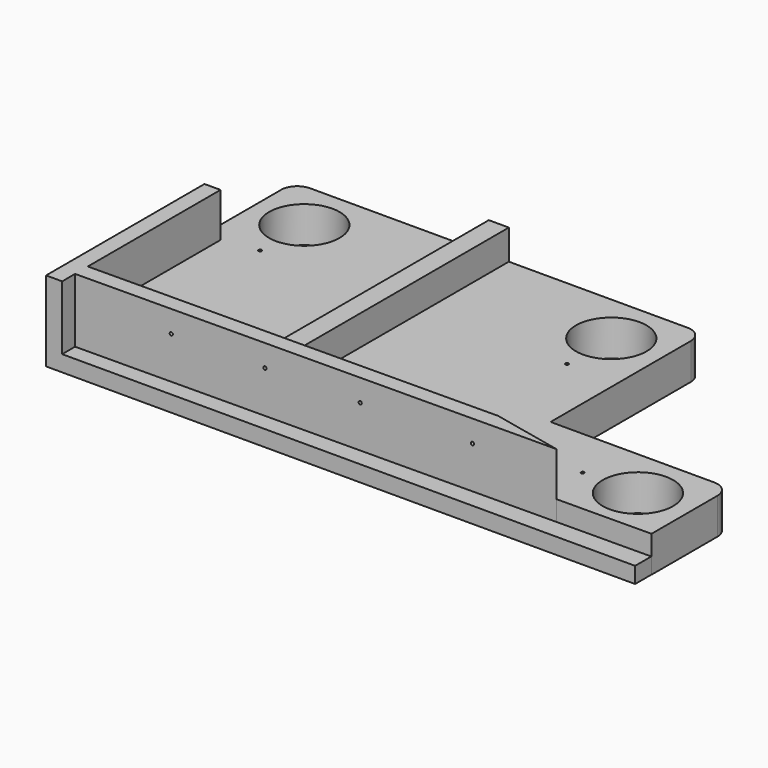
from build123d import *

# Parameters (mm, degrees)
F0_R      = 0.508
F0_R_2    = 11.176
F1_DEPTH  = 11.43
F3_DEPTH  = 25.4
F4_R      = 0.508
F5_DEPTH  = 11.4608454435
F6_W      = 6.7929165438
F6_H      = 5.08
F7_DEPTH  = 186.69
F8_W      = 6.35
F8_H      = 9.525
F9_DEPTH  = 89.916
F10_R     = 11.176
F10_R_2   = 0.508
F11_DEPTH = 5.08
F12_R     = 2.54


with BuildPart() as f1:
    # F0 (on Top) → F1 (new body)
    with BuildSketch(Plane.XY):
        with BuildLine():
            Line((9.2787205281, 23.6336458474), (9.2787205281, 79.1782657933))
            ThreePointArc((9.2787205281, 79.1782657933), (7.7908229766, 82.7703682418), (4.1987205281, 84.2582657933))
            Line((4.1987205281, 84.2582657933), (-115.4352794719, 84.2582657933))
            ThreePointArc((-115.4352794719, 84.2582657933), (-119.0273819203, 82.7703682418), (-120.5152794719, 79.1782657933))
            Line((-120.5152794719, 79.1782657933), (-120.5152794719, -8.872853592))
            Line((-120.5152794719, -8.872853592), (66.2345588207, -7.5725922361))
            Line((66.2345588207, -7.5725922361), (66.2345588207, 18.5536458474))
            ThreePointArc((66.2345588207, 18.5536458474), (64.7466612692, 22.1457482959), (61.1545588207, 23.6336458474))
            Line((61.1545588207, 23.6336458474), (9.2787205281, 23.6336458474))
        make_face()
        with Locations((32.4525588207, 7.3776458474)):
            Circle(F0_R, mode=Mode.SUBTRACT)
        with Locations((49.9785588207, 7.3776458474)):
            Circle(F0_R_2, mode=Mode.SUBTRACT)
        with Locations((-104.2592794719, 50.4762657933)):
            Circle(F0_R, mode=Mode.SUBTRACT)
        with Locations((-104.2592794719, 68.0022657933)):
            Circle(F0_R_2, mode=Mode.SUBTRACT)
        with Locations((-6.9772794719, 50.4762657933)):
            Circle(F0_R, mode=Mode.SUBTRACT)
        with Locations((-6.9772794719, 68.0022657933)):
            Circle(F0_R_2, mode=Mode.SUBTRACT)
    extrude(amount=F1_DEPTH)

    # F2 (on Top) → F3 (join)
    with BuildSketch(Plane.XY):
        Polygon((-115.4352794719, 48.7675257027), (-120.5152794719, 48.7675257027), (-120.5152794719, -13.9880853735), (-115.3984715341, -13.9880853735), (-115.4352794719, -8.872853592), (36.2575173668, -7.7813098924), (13.9111343974, -2.8922683759), (-115.4352794719, -3.792853592), align=None)
    extrude(amount=F3_DEPTH)

    # F4 (on face) → F5 (cut, through all)
    with BuildSketch(Plane(origin=(0.0208110294, -2.9889809132, 0), x_dir=(-0.9999757621, -0.0069624148, 0), z_dir=(-0.0069624148, 0.9999757621, 0))):
        with Locations((-9.7697973251, 18.415)):
            Circle(F4_R)
        with Locations((25.6308149546, 18.415)):
            Circle(F4_R)
        with Locations((55.6280761957, 18.415)):
            Circle(F4_R)
        with Locations((85.1589813828, 18.415)):
            Circle(F4_R)
    extrude(amount=-F5_DEPTH, mode=Mode.SUBTRACT)

    # F6 (on face) → F7 (join)
    with BuildSketch(Plane(origin=(-120.5152794719, 0, 0), x_dir=(0, -1, 0), z_dir=(-1, 0, 0))):
        with Locations((10.5916271016, 2.54)):
            Rectangle(F6_W, F6_H)
    extrude(amount=-F7_DEPTH)

    # F8 (on face) → F9 (join)
    with BuildSketch(Plane(origin=(0, 84.2582657933, 0), x_dir=(-1, 0, 0), z_dir=(0, 1, 0))):
        with Locations((55.6182794719, 16.1925)):
            Rectangle(F8_W, F8_H)
    extrude(amount=-F9_DEPTH)


with BuildPart() as f11:
    # F10 (on face) → F11 (new body)
    with BuildSketch(Plane(origin=(0, 0, 0), x_dir=(1, 0, 0), z_dir=(0, 0, -1))):
        with BuildLine():
            ThreePointArc((-113.3479585097, -58.1381371295), (-109.6444367223, -80.286613653), (-90.8464080064, -68.0022657933))
            ThreePointArc((-90.8464080064, -68.0022657933), (-92.1986532448, -62.1331588801), (-95.9827303886, -57.447463274))
            ThreePointArc((-95.9827303886, -57.447463274), (-99.8812141792, -55.3240299049), (-104.2592794719, -54.5893943279))
            ThreePointArc((-104.2592794719, -54.5893943279), (-109.1377439363, -55.5080389098), (-113.3479585097, -58.1381371295))
        make_face()
        with Locations((-104.2592794719, -68.0022657933)):
            Circle(F10_R, mode=Mode.SUBTRACT)
        with BuildLine():
            ThreePointArc((-104.2592794719, -54.5893943279), (-99.8812141792, -55.3240299049), (-95.9827303886, -57.447463274))
            Line((-95.9827303886, -57.447463274), (-100.364795277, -49.1530805465))
            ThreePointArc((-100.364795277, -49.1530805465), (-100.2011801378, -49.80570175), (-100.1461509373, -50.4762657933))
            ThreePointArc((-100.1461509373, -50.4762657933), (-101.3508583932, -53.384686872), (-104.2592794719, -54.5893943279))
        make_face()
        with BuildLine():
            Line((-107.8347285432, -48.4430441429), (-113.3479585097, -58.1381371295))
            ThreePointArc((-113.3479585097, -58.1381371295), (-109.1377439363, -55.5080389098), (-104.2592794719, -54.5893943279))
            ThreePointArc((-104.2592794719, -54.5893943279), (-107.8146084531, -52.5444684374), (-107.8347285432, -48.4430441429))
        make_face()
        with BuildLine():
            ThreePointArc((-107.8347285432, -48.4430441429), (-107.8146084531, -52.5444684374), (-104.2592794719, -54.5893943279))
            ThreePointArc((-104.2592794719, -54.5893943279), (-101.3508583932, -53.384686872), (-100.1461509373, -50.4762657933))
            ThreePointArc((-100.1461509373, -50.4762657933), (-100.2011801378, -49.80570175), (-100.364795277, -49.1530805465))
            Line((-100.364795277, -49.1530805465), (-100.9714052762, -48.0048877131))
            ThreePointArc((-100.9714052762, -48.0048877131), (-104.5213292601, -46.3714934184), (-107.8347285432, -48.4430441429))
        make_face()
        with Locations((-104.2592794719, -50.4762657933)):
            Circle(F10_R_2, mode=Mode.SUBTRACT)
        with Locations((-104.2592794719, -68.0022657933)):
            Circle(F10_R)
    extrude(amount=F11_DEPTH)

    # F12
    f12_edges = [f11.edges().sort_by_distance(p)[0] for p in [
        (-103.726226, 81.404541, -5.08),
        (-98.477068, 52.726175, -5.08),
        (-110.591344, 53.290591, -5.08),
        (-104.521329, 46.371493, -5.08),
    ]]
    fillet(f12_edges, radius=F12_R)


solid = Compound([f1.part, f11.part])
